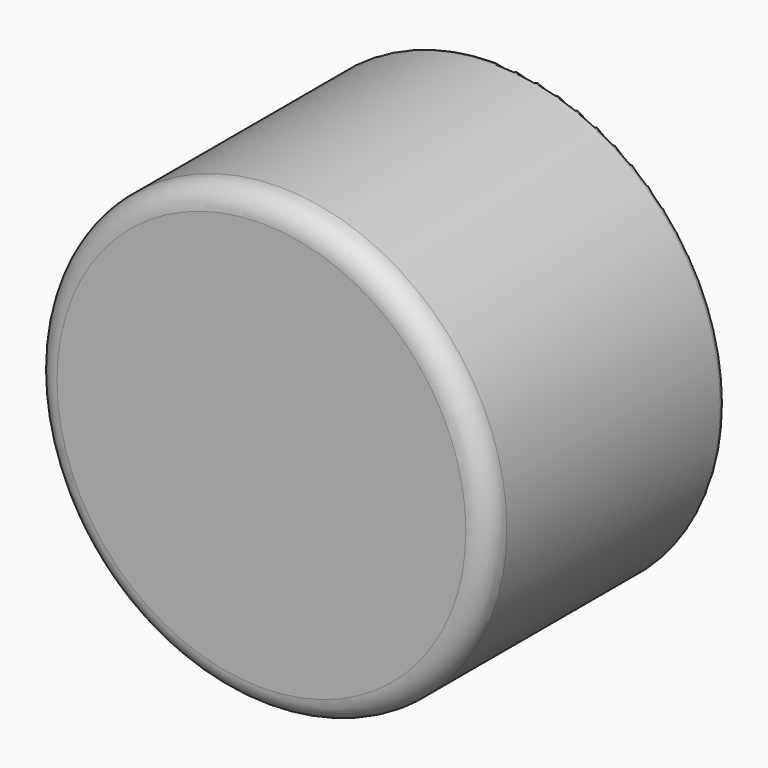
from build123d import *

# Parameters (mm, degrees)
F2_R = 5.08
F3_R = 1.27
F5_R = 1.27


# Not quite as in the source:
# - a fillet or chamfer that OpenCascade refuses, or shapes differently, is made with other operations: its cross-section is extruded or revolved along the edge and cut away or added


with BuildPart() as f1:
    # F0 (on Top) → F1 (revolve)
    with BuildSketch(Plane.XY):
        Polygon((6.35, 0), (0, 0), (0, -2.54), (50.8, -2.54), (50.8, 63.5), (48.26, 63.5), (48.26, 0), align=None)
        Polygon((0, 34.29), (0, 0), (6.35, 0), (6.35, 31.75), (19.05, 31.75), (19.05, 38.1), (16.51, 38.1), (16.51, 34.29), align=None)
    revolve(axis=Axis((0, 15.875, 0), (0, -1, 0)))

    # F2
    f2_edges = [f1.edges().sort_by_distance(p)[0] for p in [
        (-50.8, -2.54, 0),
    ]]
    fillet(f2_edges, radius=F2_R)

    # F3
    f3_edges = [f1.edges().sort_by_distance(p)[0] for p in [
        (-50.8, 63.5, 0),
    ]]
    fillet(f3_edges, radius=F3_R)

    # F4: fillet of radius 5.08 on 1 edges, made by hand

    # F4_s1 → F4_t2 (revolve, cut)
    with BuildSketch(Plane.XY):
        with BuildLine():
            ThreePointArc((49.53, 63.5), (48.5880951188, 61.9359470592), (48.26, 60.1398958349))
            Line((48.26, 60.1398958349), (48.1584, 60.1398958349))
            Line((48.1584, 60.1398958349), (48.1584, 63.5))
            Line((48.1584, 63.5), (48.26, 63.6016))
            ThreePointArc((48.26, 63.6016), (48.895, 63.6016), (49.4538, 63.5672020833))
            Line((49.4538, 63.5672020833), (49.53, 63.5))
        make_face()
    revolve(axis=Axis((0, 63.5, 0), (0, -1, 0)), mode=Mode.SUBTRACT)

    # F5
    f5_edges = [f1.edges().sort_by_distance(p)[0] for p in [
        (-19.05, 38.1, 0),
    ]]
    fillet(f5_edges, radius=F5_R)


solid = f1.part
